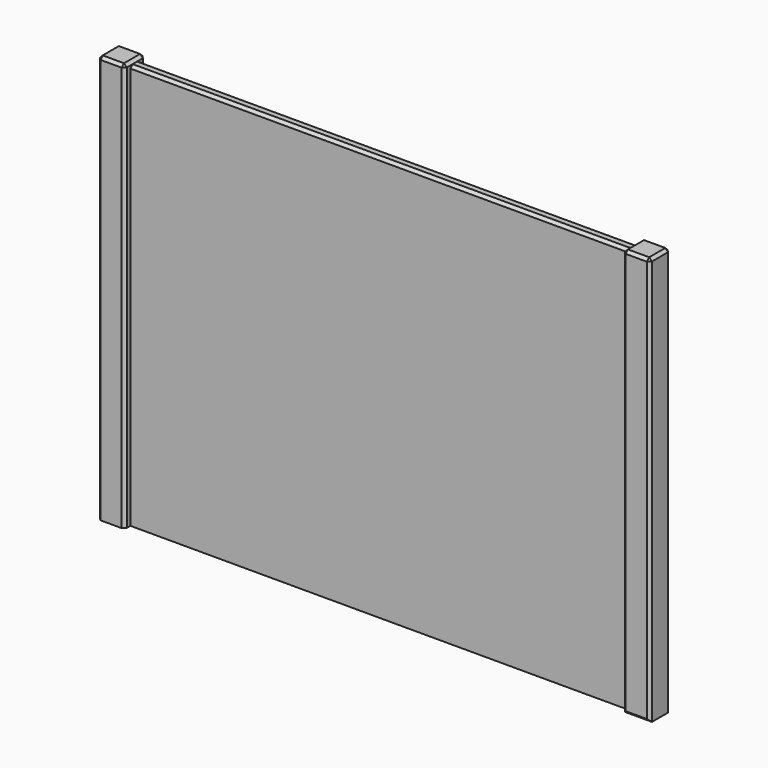
from build123d import *

# Parameters (mm, degrees)
F0_W     = 890
F0_H     = 724
F1_DEPTH = 20
F2_W     = 20
F2_H     = 724
F3_DEPTH = 48
F4_W     = 20
F4_H     = 724
F5_DEPTH = 48
F6_SIZE  = 4.9999


# Not quite as in the source:
# - a fillet or chamfer is up to 0.001 mm smaller than in the source, because OpenCascade refuses the exact size


with BuildPart() as f1:
    # F0 (on Front) → F1 (new body)
    with BuildSketch(Plane.XZ):
        with Locations((5.1721642405, -1.2866072357)):
            Rectangle(F0_W, F0_H)
    extrude(amount=F1_DEPTH)

    # F2 (on face) → F3 (join)
    with BuildSketch(Plane(origin=(-439.8278357595, 0, 0), x_dir=(0, -1, 0), z_dir=(-1, 0, 0))):
        Polygon((33, 365.7133927643), (-13, 365.7133927643), (-13, -363.2866072357), (0, -363.2866072357), (0, 360.7133927643), (20, 360.7133927643), (20, -363.2866072357), (33, -363.2866072357), align=None)
        with Locations((10, -1.2866072357)):
            Rectangle(F2_W, F2_H)
    extrude(amount=F3_DEPTH)

    # F4 (on face) → F5 (join)
    with BuildSketch(Plane.YZ.offset(450.1721642405)):
        with Locations((-10, -1.2866072357)):
            Rectangle(F4_W, F4_H)
        Polygon((13, 365.7133927643), (-33, 365.7133927643), (-33, -363.2866072357), (-20, -363.2866072357), (-20, 360.7133927643), (0, 360.7133927643), (0, -363.2866072357), (13, -363.2866072357), align=None)
    extrude(amount=F5_DEPTH)

    # F6 (size 5 in the source; OpenCascade refuses exactly that, so slightly less here)
    f6_edges = [f1.edges().sort_by_distance(p)[0] for p in [
        (-463.827836, -33, 365.713393),
        (-487.827836, -10, 365.713393),
        (-439.827836, -10, 365.713393),
        (-463.827836, 13, 365.713393),
        (5.172164, -20, 360.713393),
        (5.172164, 0, 360.713393),
        (474.172164, 13, 365.713393),
        (450.172164, -10, 365.713393),
        (474.172164, -33, 365.713393),
        (498.172164, -10, 365.713393),
        (-487.827836, 13, 1.213393),
        (-439.827836, 13, 1.213393),
        (-487.827836, -33, 1.213393),
        (-439.827836, -33, 1.213393),
        (450.172164, -33, 1.213393),
        (474.172164, -33, -363.286607),
        (498.172164, -33, 1.213393),
        (450.172164, 13, 1.213393),
        (498.172164, 13, 1.213393),
    ]]
    chamfer(f6_edges, length=F6_SIZE)


solid = f1.part
